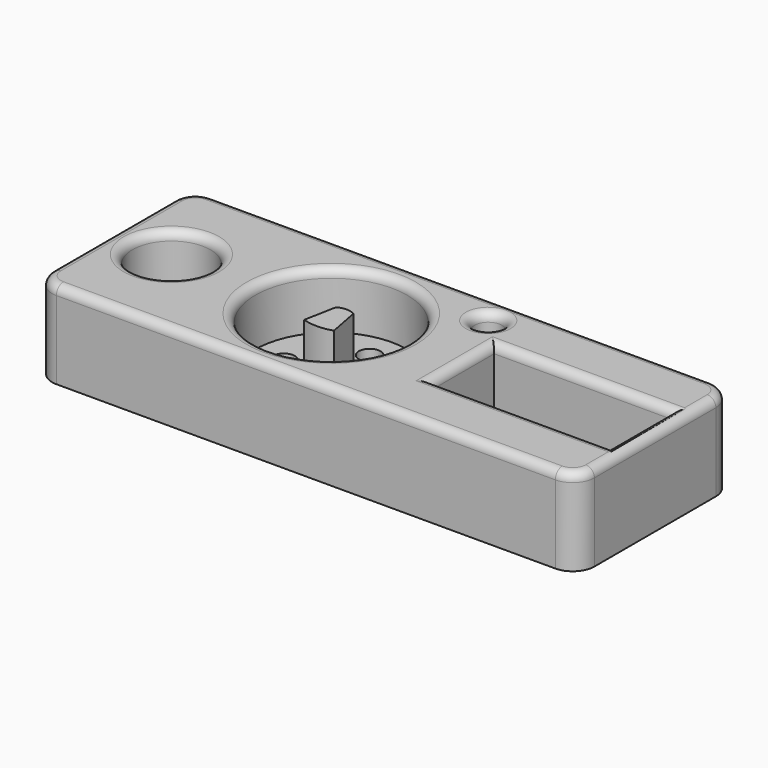
from build123d import *

# Parameters (mm, degrees)
F1_DEPTH      = 20
F3_R          = 9
F4_DEPTH      = 18
F5_R          = 17.5
F6_DEPTH      = 13
F8_DEPTH      = 12
F10_DEPTH     = 15
F11_R         = 3.15
F12_DEPTH     = 17
F13_R         = 5
F14_T1_DEPTH  = 35
F14_T3_DEPTH  = 115
F14_T5_DEPTH  = 41
F14_T7_DEPTH  = 18
F14_T10_ANGLE = 90
F14_T12_ANGLE = 90
F14_T14_ANGLE = 90
F14_T16_ANGLE = 90
F14_T27_DEPTH = 46
F14_T31_DEPTH = 23
F14_T38_DEPTH = 46
F14_T42_DEPTH = 23
F14_T49_DEPTH = 23
F14_T53_DEPTH = 46
F14_T60_DEPTH = 23
F14_T64_DEPTH = 46
F15_R         = 2.5
F16_DEPTH     = 25
F17_R         = 2.5
F18_DEPTH     = 25
F19_R         = 2
F20_DEPTH     = 25
F21_R         = 2.5
F22_DEPTH     = 25


# Not quite as in the source:
# - a fillet or chamfer that OpenCascade refuses, or shapes differently, is made with other operations: its cross-section is extruded or revolved along the edge and cut away or added
# - a feature names something its author has since deleted; it is built from what else it names


with BuildPart() as f1:
    # F0 (on Top) → F1 (new body)
    with BuildSketch(Plane.XY):
        Polygon((-50.3401843222, 22.5), (-50.3401843222, 0), (-50.3401843222, -22.5), (74.6598156778, -22.5), (74.6598156778, 22.5), align=None)
    extrude(amount=F1_DEPTH)

    # F3 (on offset) → F4 (cut)
    with BuildSketch(Plane.XY.offset(20)):
        with Locations((-36.838578499, 0)):
            Circle(F3_R)
    extrude(amount=-F4_DEPTH, mode=Mode.SUBTRACT)

    # F5 (on face) → F6 (cut)
    with BuildSketch(Plane.XY.offset(20)):
        Circle(F5_R)
    extrude(amount=-F6_DEPTH, mode=Mode.SUBTRACT)

    # F7 (on face) → F8 (join)
    with BuildSketch(Plane.XY.offset(7)):
        with BuildLine():
            Line((3.4091057572, -3.4919061418), (2, 3.8745326834))
            ThreePointArc((2, 3.8745326834), (0.0310836546, 4.3983310157), (-1.9455862415, 3.9045978994))
            ThreePointArc((-1.9455862415, 3.9045978994), (-1.9886724642, 3.8669361828), (-2.0114917871, 3.8144566059))
            Line((-2.0114917871, 3.8144566059), (-3.4205975443, -3.5519822192))
            ThreePointArc((-3.4205975443, -3.5519822192), (-0.0011175453, -4.0481144365), (3.4091057572, -3.4919061418))
        make_face()
    extrude(amount=F8_DEPTH)

    # F9 (on face) → F10 (cut)
    with BuildSketch(Plane.XY.offset(20)):
        Polygon((30.3623908478, 9), (30.3623908478, 0), (30.3623908478, -9), (71.3623908478, -9), (71.3623908478, 0), (71.3623908478, 9), align=None)
    extrude(amount=-F10_DEPTH, mode=Mode.SUBTRACT)

    # F11 (on face) → F12 (cut)
    with BuildSketch(Plane.XY.offset(20)):
        with Locations((23.8011702895, 15.4771208763)):
            Circle(F11_R)
    extrude(amount=-F12_DEPTH, mode=Mode.SUBTRACT)

    # F13
    f13_edges = [f1.edges().sort_by_distance(p)[0] for p in [
        (74.659816, -22.5, 10),
        (74.659816, 22.5, 10),
        (-50.340184, -22.5, 10),
        (-50.340184, 22.5, 10),
    ]]
    fillet(f13_edges, radius=F13_R)

    # F14: fillet of radius 2 on 15 edges, made by hand

    # F14_s2 → F14_t1 (cut)
    with BuildSketch(Plane.XZ.offset(-17.5)):
        with BuildLine():
            ThreePointArc((-50.3401843222, 18), (-49.7543978846, 19.4142135624), (-48.3401843222, 20))
            Line((-48.3401843222, 20), (-50.3401843222, 20))
            Line((-50.3401843222, 20), (-50.3401843222, 18))
        make_face()
        with BuildLine():
            ThreePointArc((72.6598156778, 20), (74.0740292402, 19.4142135624), (74.6598156778, 18))
            Line((74.6598156778, 18), (74.6598156778, 20))
            Line((74.6598156778, 20), (72.6598156778, 20))
        make_face()
    extrude(amount=F14_T1_DEPTH, mode=Mode.SUBTRACT)

    # F14_s4 → F14_t3 (cut)
    with BuildSketch(Plane.YZ.offset(-45.3401843222)):
        with BuildLine():
            ThreePointArc((-20.5, 20), (-21.9142135624, 19.4142135624), (-22.5, 18))
            Line((-22.5, 18), (-22.5, 20))
            Line((-22.5, 20), (-20.5, 20))
        make_face()
        with BuildLine():
            ThreePointArc((20.5, 20), (21.9142135624, 19.4142135624), (22.5, 18))
            Line((22.5, 18), (22.5, 20))
            Line((22.5, 20), (20.5, 20))
        make_face()
    extrude(amount=F14_T3_DEPTH, mode=Mode.SUBTRACT)

    # F14_s6 → F14_t5 (cut)
    with BuildSketch(Plane.YZ.offset(30.3623908478)):
        with BuildLine():
            ThreePointArc((-11, 20), (-9.5857864376, 19.4142135624), (-9, 18))
            Line((-9, 18), (-9, 20))
            Line((-9, 20), (-11, 20))
        make_face()
        with BuildLine():
            ThreePointArc((11, 20), (9.5857864376, 19.4142135624), (9, 18))
            Line((9, 18), (9, 20))
            Line((9, 20), (11, 20))
        make_face()
    extrude(amount=F14_T5_DEPTH, mode=Mode.SUBTRACT)

    # F14_s8 → F14_t7 (cut)
    with BuildSketch(Plane.XZ.offset(-9)):
        with BuildLine():
            ThreePointArc((28.3623908478, 20), (29.7766044102, 19.4142135624), (30.3623908478, 18))
            Line((30.3623908478, 18), (30.3623908478, 20))
            Line((30.3623908478, 20), (28.3623908478, 20))
        make_face()
        with BuildLine():
            ThreePointArc((73.3623908478, 20), (71.9481772854, 19.4142135624), (71.3623908478, 18))
            Line((71.3623908478, 18), (71.3623908478, 20))
            Line((71.3623908478, 20), (73.3623908478, 20))
        make_face()
    extrude(amount=F14_T7_DEPTH, mode=Mode.SUBTRACT)

    # F14_s9 → F14_t10 (revolve, cut)
    with BuildSketch(Plane.XZ.offset(17.5)):
        with BuildLine():
            ThreePointArc((-48.3401843222, 20), (-49.7543978846, 19.4142135624), (-50.3401843222, 18))
            Line((-50.3401843222, 18), (-50.3401843222, 20))
            Line((-50.3401843222, 20), (-48.3401843222, 20))
        make_face()
    revolve(axis=Axis((-45.3401843222, -17.5, 20), (0, 0, 1)), revolution_arc=F14_T10_ANGLE, mode=Mode.SUBTRACT)

    # F14_s11 → F14_t12 (revolve, cut)
    with BuildSketch(Plane.XZ.offset(-17.5)):
        with BuildLine():
            ThreePointArc((-48.3401843222, 20), (-49.7543978846, 19.4142135624), (-50.3401843222, 18))
            Line((-50.3401843222, 18), (-50.3401843222, 20))
            Line((-50.3401843222, 20), (-48.3401843222, 20))
        make_face()
    revolve(axis=Axis((-45.3401843222, 17.5, 20), (0, 0, -1)), revolution_arc=F14_T12_ANGLE, mode=Mode.SUBTRACT)

    # F14_s13 → F14_t14 (revolve, cut)
    with BuildSketch(Plane.YZ.offset(69.6598156778)):
        with BuildLine():
            ThreePointArc((-20.5, 20), (-21.9142135624, 19.4142135624), (-22.5, 18))
            Line((-22.5, 18), (-22.5, 20))
            Line((-22.5, 20), (-20.5, 20))
        make_face()
    revolve(axis=Axis((69.6598156778, -17.5, 20), (0, 0, 1)), revolution_arc=F14_T14_ANGLE, mode=Mode.SUBTRACT)

    # F14_s15 → F14_t16 (revolve, cut)
    with BuildSketch(Plane.YZ.offset(69.6598156778)):
        with BuildLine():
            ThreePointArc((20.5, 20), (21.9142135624, 19.4142135624), (22.5, 18))
            Line((22.5, 18), (22.5, 20))
            Line((22.5, 20), (20.5, 20))
        make_face()
    revolve(axis=Axis((69.6598156778, 17.5, 20), (0, 0, -1)), revolution_arc=F14_T16_ANGLE, mode=Mode.SUBTRACT)

    # F14_s17 → F14_t18 (revolve, cut)
    with BuildSketch(Plane.XZ):
        with BuildLine():
            ThreePointArc((-25.838578499, 20), (-27.2527920613, 19.4142135624), (-27.838578499, 18))
            Line((-27.838578499, 18), (-27.838578499, 20))
            Line((-27.838578499, 20), (-25.838578499, 20))
        make_face()
    revolve(axis=Axis((-36.838578499, 0, 20), (0, 0, 1)), mode=Mode.SUBTRACT)

    # F14_s19 → F14_t20 (revolve, cut)
    with BuildSketch(Plane.XZ):
        with BuildLine():
            ThreePointArc((19.5, 20), (18.0857864376, 19.4142135624), (17.5, 18))
            Line((17.5, 18), (17.5, 20))
            Line((17.5, 20), (19.5, 20))
        make_face()
    revolve(axis=Axis((0, 0, 20), (0, 0, 1)), mode=Mode.SUBTRACT)

    # F14_s21 → F14_t22 (revolve, cut)
    with BuildSketch(Plane.XZ.offset(-15.4771208763)):
        with BuildLine():
            ThreePointArc((28.9511702895, 20), (27.5369567271, 19.4142135624), (26.9511702895, 18))
            Line((26.9511702895, 18), (26.9511702895, 20))
            Line((26.9511702895, 20), (28.9511702895, 20))
        make_face()
    revolve(axis=Axis((23.8011702895, 15.4771208763, 20), (0, 0, 1)), mode=Mode.SUBTRACT)


with BuildPart() as f14_tool25:
    # F14_s26 → F14_t27 (new body)
    with BuildSketch(Plane.YZ.offset(25.3623908478)):
        with BuildLine():
            ThreePointArc((-11, 20), (-9.5857864376, 19.4142135624), (-9, 18))
            Line((-9, 18), (-9, 20))
            Line((-9, 20), (-11, 20))
        make_face()
    extrude(amount=F14_T27_DEPTH)

    split(bisect_by=Plane.YZ.offset(30.3623908478), keep=Keep.BOTTOM)


with BuildPart() as f14_tool29:
    # F14_s30 → F14_t31 (new body)
    with BuildSketch(Plane.XZ.offset(14)):
        with BuildLine():
            ThreePointArc((28.3623908478, 20), (29.7766044102, 19.4142135624), (30.3623908478, 18))
            Line((30.3623908478, 18), (30.3623908478, 20))
            Line((30.3623908478, 20), (28.3623908478, 20))
        make_face()
    extrude(amount=-F14_T31_DEPTH)

    split(bisect_by=Plane.XZ.offset(9), keep=Keep.TOP)


with BuildPart() as f14_tool25_1:
    add(f14_tool25.part)

    # F14_t33: intersect F14_tool29
    add(f14_tool29.part, mode=Mode.INTERSECT)


with BuildPart() as f1_1:
    add(f1.part)

    # F14_t23: cut F14_tool25
    add(f14_tool25_1.part, mode=Mode.SUBTRACT)


with BuildPart() as f14_tool36:
    # F14_s37 → F14_t38 (new body)
    with BuildSketch(Plane.YZ.offset(30.3623908478)):
        with BuildLine():
            ThreePointArc((-11, 20), (-9.5857864376, 19.4142135624), (-9, 18))
            Line((-9, 18), (-9, 20))
            Line((-9, 20), (-11, 20))
        make_face()
    extrude(amount=F14_T38_DEPTH)

    split(bisect_by=Plane.YZ.offset(71.3623908478), keep=Keep.TOP)


with BuildPart() as f14_tool40:
    # F14_s41 → F14_t42 (new body)
    with BuildSketch(Plane.XZ.offset(-9)):
        with BuildLine():
            ThreePointArc((73.3623908478, 20), (71.9481772854, 19.4142135624), (71.3623908478, 18))
            Line((71.3623908478, 18), (71.3623908478, 20))
            Line((71.3623908478, 20), (73.3623908478, 20))
        make_face()
    extrude(amount=F14_T42_DEPTH)

    split(bisect_by=Plane.XZ.offset(9), keep=Keep.TOP)


with BuildPart() as f14_tool36_1:
    add(f14_tool36.part)

    # F14_t44: intersect F14_tool40
    add(f14_tool40.part, mode=Mode.INTERSECT)


with BuildPart() as f1_2:
    add(f1_1.part)

    # F14_t34: cut F14_tool36
    add(f14_tool36_1.part, mode=Mode.SUBTRACT)


with BuildPart() as f14_tool47:
    # F14_s48 → F14_t49 (new body)
    with BuildSketch(Plane.XZ.offset(9)):
        with BuildLine():
            ThreePointArc((28.3623908478, 20), (29.7766044102, 19.4142135624), (30.3623908478, 18))
            Line((30.3623908478, 18), (30.3623908478, 20))
            Line((30.3623908478, 20), (28.3623908478, 20))
        make_face()
    extrude(amount=-F14_T49_DEPTH)

    split(bisect_by=Plane.XZ.offset(-9), keep=Keep.BOTTOM)


with BuildPart() as f14_tool51:
    # F14_s52 → F14_t53 (new body)
    with BuildSketch(Plane.YZ.offset(71.3623908478)):
        with BuildLine():
            ThreePointArc((11, 20), (9.5857864376, 19.4142135624), (9, 18))
            Line((9, 18), (9, 20))
            Line((9, 20), (11, 20))
        make_face()
    extrude(amount=-F14_T53_DEPTH)

    split(bisect_by=Plane.YZ.offset(30.3623908478), keep=Keep.BOTTOM)


with BuildPart() as f14_tool47_1:
    add(f14_tool47.part)

    # F14_t55: intersect F14_tool51
    add(f14_tool51.part, mode=Mode.INTERSECT)


with BuildPart() as f1_3:
    add(f1_2.part)

    # F14_t45: cut F14_tool47
    add(f14_tool47_1.part, mode=Mode.SUBTRACT)


with BuildPart() as f14_tool58:
    # F14_s59 → F14_t60 (new body)
    with BuildSketch(Plane.XZ.offset(-14)):
        with BuildLine():
            ThreePointArc((73.3623908478, 20), (71.9481772854, 19.4142135624), (71.3623908478, 18))
            Line((71.3623908478, 18), (71.3623908478, 20))
            Line((71.3623908478, 20), (73.3623908478, 20))
        make_face()
    extrude(amount=F14_T60_DEPTH)

    split(bisect_by=Plane.XZ.offset(-9), keep=Keep.BOTTOM)


with BuildPart() as f14_tool62:
    # F14_s63 → F14_t64 (new body)
    with BuildSketch(Plane.YZ.offset(76.3623908478)):
        with BuildLine():
            ThreePointArc((11, 20), (9.5857864376, 19.4142135624), (9, 18))
            Line((9, 18), (9, 20))
            Line((9, 20), (11, 20))
        make_face()
    extrude(amount=-F14_T64_DEPTH)

    split(bisect_by=Plane.YZ.offset(71.3623908478), keep=Keep.TOP)


with BuildPart() as f14_tool58_1:
    add(f14_tool58.part)

    # F14_t66: intersect F14_tool62
    add(f14_tool62.part, mode=Mode.INTERSECT)


with BuildPart() as f1_4:
    add(f1_3.part)

    # F14_t56: cut F14_tool58
    add(f14_tool58_1.part, mode=Mode.SUBTRACT)

    # F15 (on face) → F16 (cut)
    with BuildSketch(Plane.XY.offset(2)):
        with Locations((-36.838578499, 0)):
            Circle(F15_R)
    extrude(amount=-F16_DEPTH, mode=Mode.SUBTRACT)

    # F17 (on face) → F18 (cut)
    with BuildSketch(Plane.XY.offset(7)):
        with Locations((0, 11.0690705478)):
            Circle(F17_R)
        with Locations((-10.9194163233, 0)):
            Circle(F17_R)
        with Locations((0, -11.1288661137)):
            Circle(F17_R)
        with Locations((11.8041224778, 0)):
            Circle(F17_R)
    extrude(amount=-F18_DEPTH, mode=Mode.SUBTRACT)

    # F19 (on face) → F20 (cut)
    with BuildSketch(Plane.XY.offset(3)):
        with Locations((23.8011702895, 15.4771208763)):
            Circle(F19_R)
    extrude(amount=-F20_DEPTH, mode=Mode.SUBTRACT)

    # F21 (on face) → F22 (cut)
    with BuildSketch(Plane.XY.offset(5)):
        with Locations((36.3787501116, 0)):
            Circle(F21_R)
        with Locations((58.4114133848, 0)):
            Circle(F21_R)
    extrude(amount=-F22_DEPTH, mode=Mode.SUBTRACT)


solid = f1_4.part
